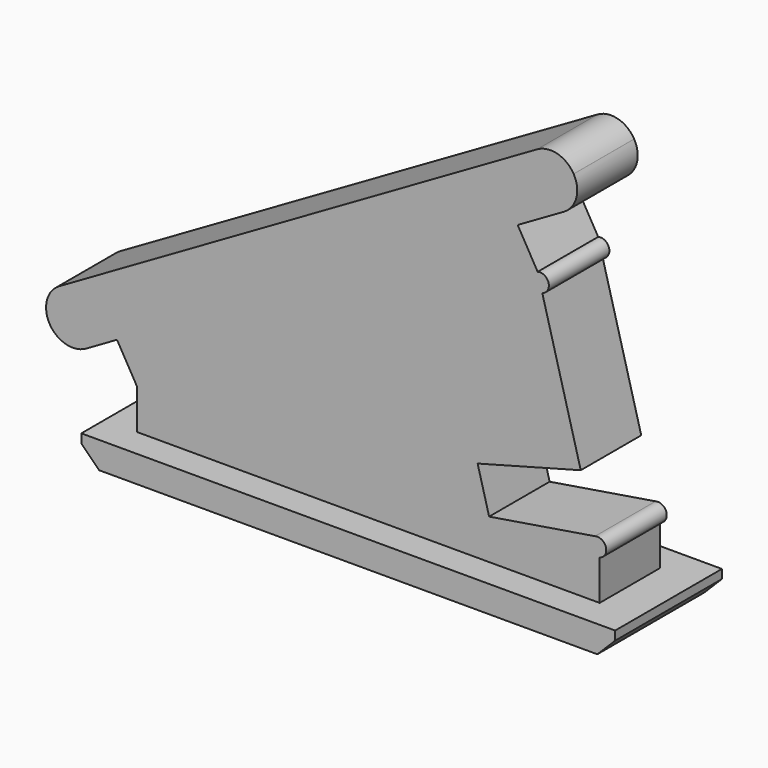
from build123d import *

# Parameters (mm, degrees)
F1_DEPTH = 3.75
F2_DEPTH = 2.125
F3_SIZE  = 1


# Not quite as in the source:
# - a feature names something its author has since deleted; it is built from what else it names


with BuildPart() as f1:
    # F0 (on Front) → F1 (new body, symmetric)
    with BuildSketch(Plane.XZ):
        Polygon((-22.420435602, 1.5), (-24.2496415957, 1.5), (-24.2496415957, 0), (5.7503584043, 0), (5.7503584043, 1.5), (3.579564398, 1.5), align=None)
    extrude(amount=F1_DEPTH, both=True)

    # F0 (on Front) → F2 (join, symmetric)
    with BuildSketch(Plane.XZ):
        with BuildLine():
            Line((-23.545435602, 5.6985571585), (-22.420435602, 3.75))
            Line((-22.420435602, 3.75), (0.0962248963, 16.75))
            Line((0.0962248963, 16.75), (-1.0287751037, 18.6985571585))
            Line((-1.0287751037, 18.6985571585), (1.5693069281, 20.1985605189))
            ThreePointArc((1.5693069281, 20.1985605189), (2.2681808156, 21.1093697133), (2.1183275727, 22.2475885433))
            Line((2.1183275727, 22.2475885433), (2.117101021, 22.2497129931))
            ThreePointArc((2.117101021, 22.2497129931), (1.2027410199, 22.9495484169), (0.0617075083, 22.7950610152))
            Line((0.0617075083, 22.7950610152), (-26.7819009783, 7.2968964295))
            ThreePointArc((-26.7819009783, 7.2968964295), (-27.4812661607, 6.3843043976), (-27.329090085, 5.2446648418))
            Line((-27.329090085, 5.2446648418), (-27.3278673466, 5.242558978))
            ThreePointArc((-27.3278673466, 5.242558978), (-26.4171243137, 4.5463872777), (-25.2806782399, 4.6967143544))
            Line((-25.2806782399, 4.6967143544), (-23.545435602, 5.6985571585))
        make_face()
        Polygon((0.0962248963, 16.75), (-22.420435602, 3.75), (-2.6320926845, 3.75), (-3.2791402973, 6.1648145657), (2.5164146605, 7.7177288363), (0.3550439415, 15.7840741737), align=None)
        Polygon((-22.420435602, 3.75), (-22.420435602, 1.5), (3.579564398, 1.5), (3.579564398, 3.75), (-2.6320926845, 3.75), align=None)
        Polygon((-2.6320926845, 3.75), (3.579564398, 3.75), (3.3207453529, 4.7159258263), align=None)
        with BuildLine():
            Line((3.3207453529, 4.7159258263), (3.579564398, 3.75))
            ThreePointArc((3.579564398, 3.75), (3.9331177885, 4.3623724357), (3.3207453529, 4.7159258263))
        make_face()
        with BuildLine():
            ThreePointArc((0.3550439415, 15.7840741737), (0.708597332, 16.3964466094), (0.0962248963, 16.75))
            Line((0.0962248963, 16.75), (0.3550439415, 15.7840741737))
        make_face()
    extrude(amount=F2_DEPTH, both=True)

    # F3
    f3_edges = [f1.edges().sort_by_distance(p)[0] for p in [
        (-24.249642, 0, 0),
        (5.750358, 0, 0),
    ]]
    chamfer(f3_edges, length=F3_SIZE)


solid = f1.part
